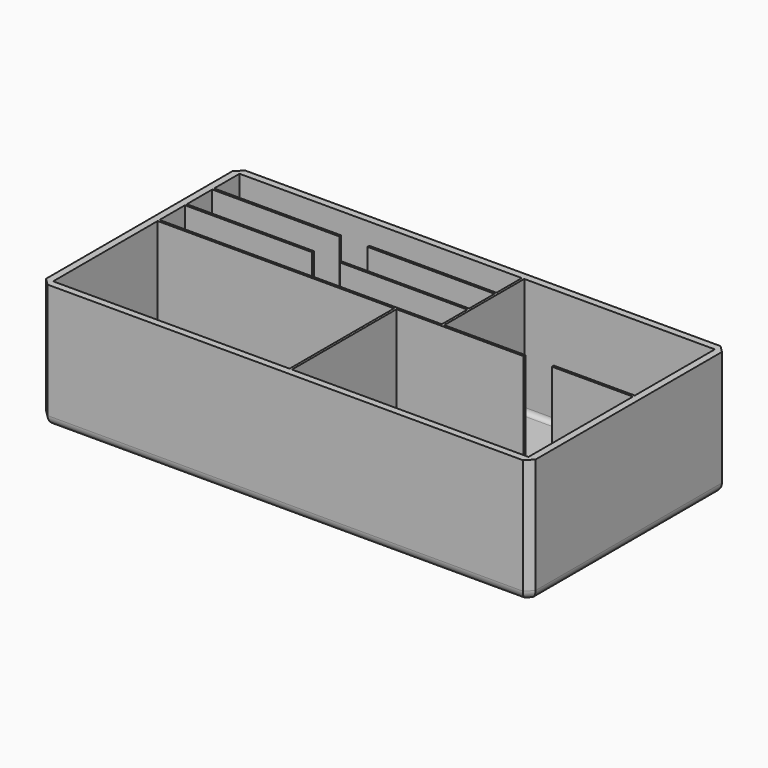
from build123d import *

# Parameters (mm, degrees)
F0_W          = 208
F0_H          = 105
F1_DEPTH      = 53
F2_T          = -3
F3_W          = 120
F3_H          = 1
F3_W_2        = 1
F3_H_2        = 13.5
F3_H_3        = 55.5
F4_DEPTH      = 50
F5_SIZE       = 3
F6_R          = 4
F7_W          = 12
F7_H          = 50
F8_DEPTH      = 10
F8_DEPTH_BACK = 15
F9_W          = 12
F9_H          = 50
F10_DEPTH     = 5
F11_R         = 2
F12_TEXT_SIZE = 32.6802808274
F13_DEPTH     = 2
F14_TEXT_SIZE = 9.5235592082
F15_DEPTH     = 2
F16_TEXT_SIZE = 8.6878097532
F17_DEPTH     = 2


# Not quite as in the source:
# - Text() gives the source's letters only with a copy of the font that has no kerning and outlines rounded to 1/6400 em; it was checked with that copy


with BuildPart() as f1:
    # F0 (on Top) → F1 (new body)
    with BuildSketch(Plane.XY):
        with Locations((61.8614929318, 37.6107571033)):
            Rectangle(F0_W, F0_H)
    extrude(amount=F1_DEPTH)

    # F2
    f2_openings = [f1.faces().sort_by_distance(p)[0] for p in [
        (61.861493, 37.610757, 53),
    ]]
    offset(amount=F2_T, openings=f2_openings)

    # F3 (on face) → F4 (join)
    with BuildSketch(Plane.XY.offset(3)):
        with Locations((20.8614929318, 73.1107571033)):
            Rectangle(F3_W, F3_H)
        with Locations((81.3614929318, 80.3607571033)):
            Rectangle(F3_W_2, F3_H_2)
        with Locations((81.3614929318, 73.1107571033)):
            Rectangle(F3_W_2, F3_H)
        with Locations((81.3614929318, 65.8607571033)):
            Rectangle(F3_W_2, F3_H_2)
        with Locations((20.8614929318, 58.6107571033)):
            Rectangle(F3_W, F3_H)
        with Locations((81.3614929318, 58.6107571033)):
            Rectangle(F3_W_2, F3_H)
        with Locations((81.3614929318, 51.3607571033)):
            Rectangle(F3_W_2, F3_H_2)
        Polygon((81.8614929318, 44.6107571033), (80.8614929318, 44.6107571033), (-39.1385070682, 44.6107571033), (-39.1385070682, 43.6107571033), (61.3614929318, 43.6107571033), (62.3614929318, 43.6107571033), (162.8614929318, 43.6107571033), (162.8614929318, 44.6107571033), align=None)
        with Locations((61.8614929318, 15.8607571033)):
            Rectangle(F3_W_2, F3_H_3)
    extrude(amount=F4_DEPTH)

    # F5
    f5_edges = [f1.edges().sort_by_distance(p)[0] for p in [
        (165.861493, -14.889243, 26.5),
        (165.861493, 90.110757, 26.5),
        (-42.138507, -14.889243, 26.5),
        (-42.138507, 90.110757, 26.5),
    ]]
    chamfer(f5_edges, length=F5_SIZE)

    # F6
    f6_edges = [f1.edges().sort_by_distance(p)[0] for p in [
        (-42.138507, 37.610757, 0),
        (-40.638507, 88.610757, 0),
        (-40.638507, -13.389243, 0),
        (61.861493, 90.110757, 0),
        (61.861493, -14.889243, 0),
        (164.361493, 88.610757, 0),
        (164.361493, -13.389243, 0),
        (165.861493, 37.610757, 0),
    ]]
    fillet(f6_edges, radius=F6_R)

    # F7 (on face) → F8 (cut, two sides)
    with BuildSketch(Plane.XZ.offset(-72.6107571033)) as f8_sk:
        with Locations((20.8614929318, 28)):
            Rectangle(F7_W, F7_H)
    extrude(amount=-F8_DEPTH, mode=Mode.SUBTRACT)
    extrude(f8_sk.sketch, amount=F8_DEPTH_BACK, mode=Mode.SUBTRACT)

    # F9 (on face) → F10 (cut)
    with BuildSketch(Plane(origin=(0, 44.6107571033, 0), x_dir=(-1, 0, 0), z_dir=(0, 1, 0))):
        with Locations((-122.3614929318, 28)):
            Rectangle(F9_W, F9_H)
    extrude(amount=-F10_DEPTH, mode=Mode.SUBTRACT)

    # F11
    f11_edges = [f1.edges().sort_by_distance(p)[0] for p in [
        (11.111493, 43.610757, 3),
        (61.361493, 15.860757, 3),
        (11.111493, -11.889243, 3),
        (-39.138507, 15.860757, 3),
        (112.611493, -11.889243, 3),
        (162.861493, 15.860757, 3),
        (145.611493, 43.610757, 3),
        (128.361493, 44.110757, 3),
        (145.611493, 44.610757, 3),
        (162.861493, 65.860757, 3),
        (122.361493, 87.110757, 3),
        (81.861493, 65.860757, 3),
        (99.111493, 44.610757, 3),
        (116.361493, 44.110757, 3),
        (89.361493, 43.610757, 3),
        (62.361493, 15.860757, 3),
        (80.861493, 80.360757, 3),
        (20.861493, 87.110757, 3),
        (-39.138507, 80.360757, 3),
        (-12.138507, 73.610757, 3),
        (14.861493, 73.110757, 3),
        (-12.138507, 72.610757, 3),
        (-39.138507, 65.860757, 3),
        (-12.138507, 59.110757, 3),
        (14.861493, 58.610757, 3),
        (-12.138507, 58.110757, 3),
        (-39.138507, 51.360757, 3),
        (20.861493, 44.610757, 3),
        (80.861493, 51.360757, 3),
        (53.861493, 58.110757, 3),
        (26.861493, 58.610757, 3),
        (53.861493, 59.110757, 3),
        (80.861493, 65.860757, 3),
        (53.861493, 72.610757, 3),
        (26.861493, 73.110757, 3),
        (53.861493, 73.610757, 3),
    ]]
    fillet(f11_edges, radius=F11_R)

    # F12 (on face) → F13 (cut)
    with BuildSketch(Plane(origin=(0, 0, 0), x_dir=(1, 0, 0), z_dir=(0, 0, -1))):
        with Locations((-24.5397971012, -30.6739609018)):
            Text('v1.1', F12_TEXT_SIZE, font='Open Sans', text_align=(TextAlign.LEFT, TextAlign.BOTTOM))
    extrude(amount=-F13_DEPTH, mode=Mode.SUBTRACT)

    # F14 (on face) → F15 (cut)
    with BuildSketch(Plane.XY.offset(3)):
        with Locations((107.6008155942, 69.5459585997)):
            Text('ExPen', F14_TEXT_SIZE, font='Open Sans', text_align=(TextAlign.LEFT, TextAlign.BOTTOM))
        with Locations((107.6008155942, 56.5939180766)):
            Text('Papers', F14_TEXT_SIZE, font='Open Sans', text_align=(TextAlign.LEFT, TextAlign.BOTTOM))
    extrude(amount=-F15_DEPTH, mode=Mode.SUBTRACT)

    # F16 (on face) → F17 (cut)
    with BuildSketch(Plane.XY.offset(3)):
        with Locations((6.4230682328, 62.9209740297)):
            Text('ExPens', F16_TEXT_SIZE, font='Open Sans', text_align=(TextAlign.LEFT, TextAlign.BOTTOM))
    extrude(amount=-F17_DEPTH, mode=Mode.SUBTRACT)


solid = f1.part
